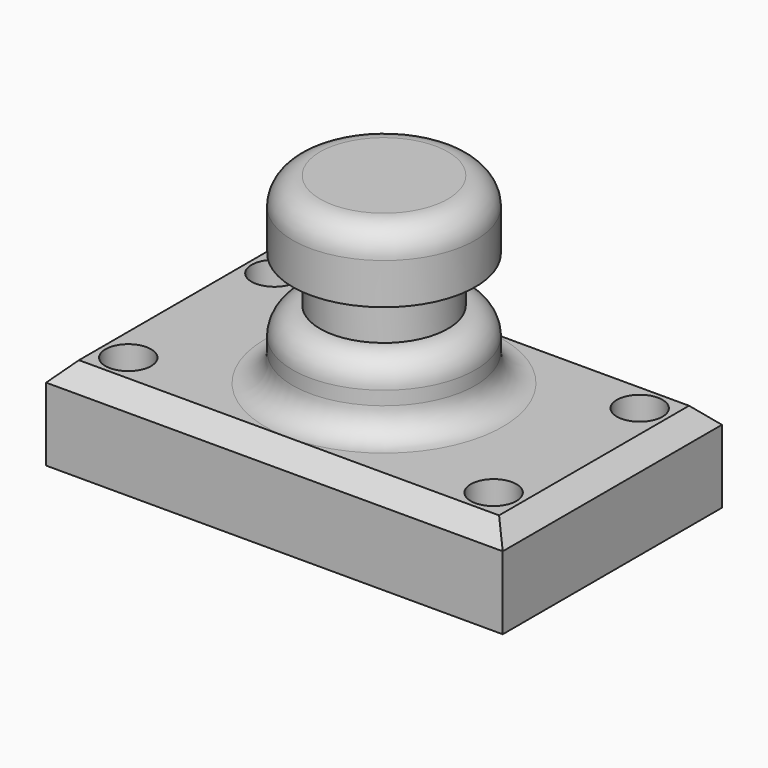
from build123d import *

# Parameters (mm, degrees)
F0_W     = 127
F0_H     = 76.2
F1_DEPTH = 12.7
F2_R     = 6.35
F3_DEPTH = 38.1
F4_W     = 25.4
F4_H     = 50.8
F6_W     = 16.0364900438
F6_H     = 12.7
F8_SIZE  = 5.08
F9_R     = 7.61999


# Not quite as in the source:
# - a fillet or chamfer is up to 0.001 mm smaller than in the source, because OpenCascade refuses the exact size


with BuildPart() as f1:
    # F0 (on Top) → F1 (new body, symmetric)
    with BuildSketch(Plane.XY):
        Rectangle(F0_W, F0_H)
    extrude(amount=F1_DEPTH, both=True)

    # F2 (on face) → F3 (cut)
    with BuildSketch(Plane.XY.offset(12.7)):
        with Locations((-50.8, 25.4)):
            Circle(F2_R)
        with Locations((50.8, 25.4)):
            Circle(F2_R)
        with Locations((50.8, -25.4)):
            Circle(F2_R)
        with Locations((-50.8, -25.4)):
            Circle(F2_R)
    extrude(amount=-F3_DEPTH, mode=Mode.SUBTRACT)

    # F4 (on Front) → F5 (revolve)
    with BuildSketch(Plane.XZ):
        with Locations((-12.7, 38.1)):
            Rectangle(F4_W, F4_H)
    revolve(axis=Axis((0, 0, 38.1), (0, 0, 1)))

    # F6 (on Front) → F7 (revolve, cut)
    with BuildSketch(Plane.XZ):
        with Locations((-25.7982450219, 38.1)):
            Rectangle(F6_W, F6_H)
    revolve(axis=Axis((0, 0, 63.5), (0, 0, -1)), mode=Mode.SUBTRACT)

    # F8
    f8_edges = [f1.edges().sort_by_distance(p)[0] for p in [
        (0, -38.1, 12.7),
        (-63.5, 0, 12.7),
        (0, 38.1, 12.7),
        (63.5, 0, 12.7),
    ]]
    chamfer(f8_edges, length=F8_SIZE)

    # F9 (radius 7.62 in the source; OpenCascade refuses exactly that, so slightly less here)
    f9_edges = [f1.edges().sort_by_distance(p)[0] for p in [
        (25.4, 0, 12.7),
        (25.4, 0, 31.75),
        (25.4, 0, 63.5),
    ]]
    fillet(f9_edges, radius=F9_R)


solid = f1.part
